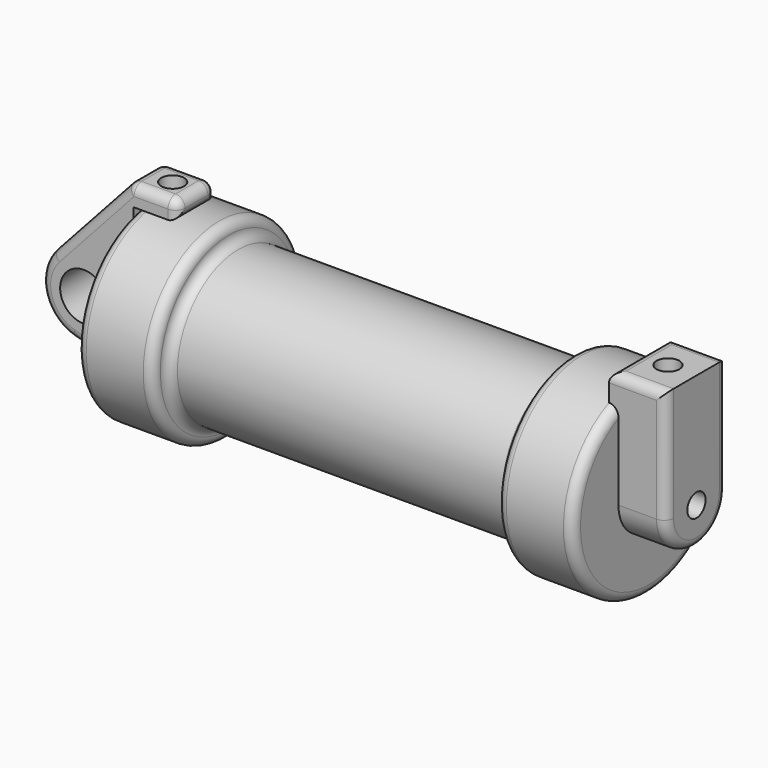
from build123d import *

# Parameters (mm, degrees)
F0_W     = 5.842
F0_H     = 12.7
F0_R     = 3.175
F2_DEPTH = 3.175
F3_R     = 1.524
F4_DEPTH = 56.134
F5_DEPTH = 6.35
F6_DEPTH = 1.27
F7_R     = 1.524
F8_DEPTH = 17.78
F9_DEPTH = 10.414
F10_R    = 1.27
F11_R    = 1.26999
F11_2_R  = 1.26999
F12_R    = 1.26999


# Not quite as in the source:
# - a fillet or chamfer is up to 0.001 mm smaller than in the source, because OpenCascade refuses the exact size


with BuildPart() as f1:
    # F0 (on Front) → F1 (revolve)
    with BuildSketch(Plane.XZ):
        Polygon((5.842, 12.7), (5.842, 0), (66.294, 0), (66.294, 12.7), (56.134, 12.7), (56.134, 10.16), (10.16, 10.16), (10.16, 12.7), align=None)
        with Locations((2.921, 6.35)):
            Rectangle(F0_W, F0_H)
    revolve(axis=Axis((33.147, 0, 0), (-1, 0, 0)))

    # F3 (on face) → F4 (cut, through all)
    with BuildSketch(Plane.YZ.offset(66.294)):
        Circle(F3_R)
    extrude(amount=-F4_DEPTH, mode=Mode.SUBTRACT)

    # F3 (on face) → F5 (join)
    with BuildSketch(Plane.YZ.offset(66.294)):
        with BuildLine():
            ThreePointArc((-5.08, 11.6397422652), (0, 12.7), (5.08, 11.6397422652))
            Line((5.08, 11.6397422652), (5.08, 15.24))
            Line((5.08, 15.24), (-5.08, 15.24))
            Line((-5.08, 15.24), (-5.08, 11.6397422652))
        make_face()
        with BuildLine():
            ThreePointArc((-5.08, 0), (0, 5.08), (5.08, 0))
            Line((5.08, 0), (5.08, 11.6397422652))
            ThreePointArc((5.08, 11.6397422652), (0, 12.7), (-5.08, 11.6397422652))
            Line((-5.08, 11.6397422652), (-5.08, 0))
        make_face()
        with BuildLine():
            ThreePointArc((-5.08, 0), (0, -5.08), (5.08, 0))
            ThreePointArc((5.08, 0), (0, 5.08), (-5.08, 0))
        make_face()
        Circle(F3_R, mode=Mode.SUBTRACT)
    extrude(amount=F5_DEPTH)

    # F3 (on face) → F6 (join)
    with BuildSketch(Plane.YZ.offset(66.294)):
        with BuildLine():
            ThreePointArc((-5.08, 11.6397422652), (0, 12.7), (5.08, 11.6397422652))
            Line((5.08, 11.6397422652), (5.08, 15.24))
            Line((5.08, 15.24), (-5.08, 15.24))
            Line((-5.08, 15.24), (-5.08, 11.6397422652))
        make_face()
        with BuildLine():
            ThreePointArc((-5.08, 0), (0, 5.08), (5.08, 0))
            Line((5.08, 0), (5.08, 11.6397422652))
            ThreePointArc((5.08, 11.6397422652), (0, 12.7), (-5.08, 11.6397422652))
            Line((-5.08, 11.6397422652), (-5.08, 0))
        make_face()
        with BuildLine():
            ThreePointArc((-5.08, 0), (0, -5.08), (5.08, 0))
            ThreePointArc((5.08, 0), (0, 5.08), (-5.08, 0))
        make_face()
        Circle(F3_R, mode=Mode.SUBTRACT)
    extrude(amount=-F6_DEPTH)

    # F7 (on face) → F9 (cut)
    with BuildSketch(Plane.XY.offset(15.24)):
        with Locations((68.834, 0)):
            Circle(F7_R)
    extrude(amount=-F9_DEPTH, mode=Mode.SUBTRACT)

    # F10
    f10_edges = [f1.edges().sort_by_distance(p)[0] for p in [
        (56.134, 0, -10.16),
        (10.16, 0, -10.16),
        (33.147, 0, 10.16),
    ]]
    fillet(f10_edges, radius=F10_R)

    # F11 (radius 1.27 in the source; OpenCascade refuses exactly that, so slightly less here)
    f11_edges = [f1.edges().sort_by_distance(p)[0] for p in [
        (10.16, 0, -12.7),
        (0, 0, -12.7),
        (5.08, 0, 12.7),
    ]]
    fillet(f11_edges, radius=F11_R)

    # F12 (radius 1.27 in the source; OpenCascade refuses exactly that, so slightly less here)
    f12_edges = [f1.edges().sort_by_distance(p)[0] for p in [
        (66.294, 0, -12.7),
        (56.134, 0, -12.7),
        (68.834, -5.08, 15.24),
        (72.644, -5.08, 7.62),
        (65.024, 0, 15.24),
        (68.834, 5.08, 15.24),
        (72.644, 5.08, 7.62),
        (72.644, 0, -5.08),
    ]]
    fillet(f12_edges, radius=F12_R)


with BuildPart() as f2:
    # F0 (on Front) → F2 (new body, symmetric)
    with BuildSketch(Plane.XZ):
        with BuildLine():
            Line((-0.9398, 0), (0, 0))
            Line((0, 0), (0, 12.7))
            Line((0, 12.7), (5.842, 12.7))
            Line((5.842, 12.7), (5.842, 15.24))
            Line((5.842, 15.24), (-0.508, 15.24))
            Line((-0.508, 15.24), (-10.8806298187, 3.8475430269))
            ThreePointArc((-10.8806298187, 3.8475430269), (-4.5919612295, 5.3297205562), (-0.9398, 0))
        make_face()
        with BuildLine():
            ThreePointArc((-8.1826630726, -5.5069827884), (-3.1957909266, -4.5493385486), (-0.9398, 0))
            ThreePointArc((-0.9398, 0), (-4.5919612295, 5.3297205562), (-10.8806298187, 3.8475430269))
            ThreePointArc((-10.8806298187, 3.8475430269), (-12.1459778134, -1.5837270034), (-8.1826630726, -5.5069827884))
        make_face()
        with Locations((-6.6548, 0)):
            Circle(F0_R, mode=Mode.SUBTRACT)
        with BuildLine():
            Line((5.842, 0), (0, 0))
            Line((0, 0), (-0.9398, 0))
            ThreePointArc((-0.9398, 0), (-3.1957909266, -4.5493385486), (-8.1826630726, -5.5069827884))
            Line((-8.1826630726, -5.5069827884), (5.842, -9.398))
            Line((5.842, -9.398), (5.842, 0))
        make_face()
    extrude(amount=F2_DEPTH, both=True)

    # F7 (on face) → F8 (cut)
    with BuildSketch(Plane.XY.offset(15.24)):
        with Locations((2.667, 0)):
            Circle(F7_R)
    extrude(amount=-F8_DEPTH, mode=Mode.SUBTRACT)

    # F11#2 (radius 1.27 in the source; OpenCascade refuses exactly that, so slightly less here)
    f11_2_edges = [f2.edges().sort_by_distance(p)[0] for p in [
        (-0.508, 0, 15.24),
        (-5.694315, 3.175, 9.543772),
        (-10.88063, 0, 3.847543),
        (-5.694315, -3.175, 9.543772),
        (5.842, 0, 12.7),
        (5.842, 3.175, 13.97),
        (5.842, 0, 15.24),
        (5.842, -3.175, 13.97),
        (2.667, -3.175, 15.24),
        (2.667, 3.175, 15.24),
    ]]
    fillet(f11_2_edges, radius=F11_2_R)


solid = Compound([f1.part, f2.part])
